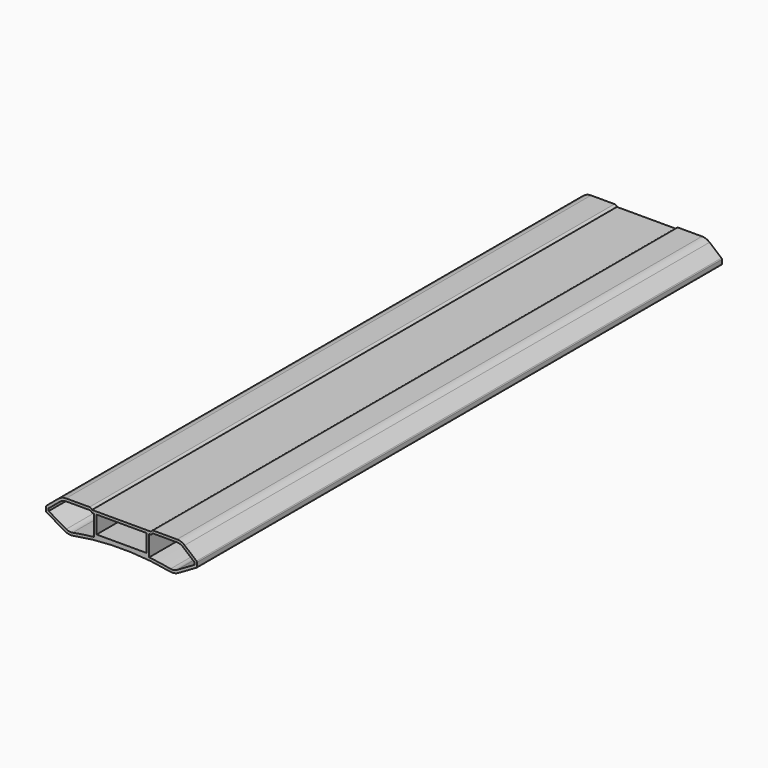
from build123d import *

# Parameters (mm, degrees)
F1_DEPTH    = 250
F2_W        = 38
F2_H        = 13.3740238536
F3_DEPTH    = 1200
F4_T1_DEPTH = 509.3674969976
F5_R        = 9
F6_R        = 1
F8_DEPTH    = 500.001


# Not quite as in the source:
# - a fillet or chamfer that OpenCascade refuses, or shapes differently, is made with other operations: its cross-section is extruded or revolved along the edge and cut away or added


with BuildPart() as f1:
    # F0 (on Front) → F1 (new body, symmetric)
    with BuildSketch(Plane.XZ):
        with BuildLine():
            Line((-57.5, 2.6740238536), (-40.1794919243, -7.3259761464))
            ThreePointArc((-40.1794919243, -7.3259761464), (0, -3.248431288), (40.1794919243, -7.3259761464))
            Line((40.1794919243, -7.3259761464), (57.5, 2.6740238536))
            Line((57.5, 2.6740238536), (57.5, 6.6740238536))
            Line((57.5, 6.6740238536), (45.5824640741, 16.6740238536))
            Line((45.5824640741, 16.6740238536), (22.5, 16.6740238536))
            Line((22.5, 16.6740238536), (22.5, 15.3740238536))
            Line((22.5, 15.3740238536), (0, 15.3740238536))
            Line((0, 15.3740238536), (-22.5, 15.3740238536))
            Line((-22.5, 15.3740238536), (-22.5, 16.6740238536))
            Line((-22.5, 16.6740238536), (-45.5824640741, 16.6740238536))
            Line((-45.5824640741, 16.6740238536), (-57.5, 6.6740238536))
            Line((-57.5, 6.6740238536), (-57.5, 2.6740238536))
        make_face()
    extrude(amount=F1_DEPTH, both=True)

    # F2 (on face) → F3 (cut)
    with BuildSketch(Plane.XZ.offset(250)):
        with Locations((0, 6.6870119268)):
            Rectangle(F2_W, F2_H)
    extrude(amount=-F3_DEPTH, mode=Mode.SUBTRACT)

    # F4: fillet of radius 2 on 2 edges, made by hand

    # F4_s2 → F4_t1 (cut)
    with BuildSketch(Plane.XZ.offset(-254.6837484988)):
        with BuildLine():
            ThreePointArc((-24.3734993995, 16.6740238536), (-23.2333239744, 16.3171915261), (-22.5, 15.3740238536))
            Line((-22.5, 15.3740238536), (-22.5, 16.6740238536))
            Line((-22.5, 16.6740238536), (-24.3734993995, 16.6740238536))
        make_face()
        with BuildLine():
            ThreePointArc((24.3734993995, 16.6740238536), (23.2333239744, 16.3171915261), (22.5, 15.3740238536))
            Line((22.5, 15.3740238536), (22.5, 16.6740238536))
            Line((22.5, 16.6740238536), (24.3734993995, 16.6740238536))
        make_face()
    extrude(amount=F4_T1_DEPTH, mode=Mode.SUBTRACT)

    # F5
    f5_edges = [f1.edges().sort_by_distance(p)[0] for p in [
        (45.582464, 0, 16.674024),
        (40.179492, 0, -7.325976),
        (-45.582464, 0, 16.674024),
        (-40.179492, 0, -7.325976),
    ]]
    fillet(f5_edges, radius=F5_R)

    # F6
    f6_edges = [f1.edges().sort_by_distance(p)[0] for p in [
        (-57.5, 0, 6.674024),
        (-57.5, 0, 2.674024),
        (57.5, 0, 6.674024),
        (57.5, 0, 2.674024),
    ]]
    fillet(f6_edges, radius=F6_R)

    # F7 (on face) → F8 (cut, through all)
    with BuildSketch(Plane.XZ.offset(250)):
        with BuildLine():
            ThreePointArc((-42.102269028, -3.9064590428), (-39.7790673217, -4.7446540804), (-37.3093701512, -4.7238460325))
            ThreePointArc((-37.3093701512, -4.7238460325), (-29.178978452, -3.3669982622), (-20.9999997169, -2.3429807302))
            Line((-20.9999997169, -2.3429807302), (-20.9999997169, 13.3740240708))
            Line((-20.9999997169, 13.3740240708), (-22.500000096, 13.3740240708))
            ThreePointArc((-22.500000096, 13.3740240708), (-23.2333241124, 14.3171915037), (-24.3734993995, 14.6740237251))
            Line((-24.3734993995, 14.6740237251), (-42.3067319657, 14.6740237251))
            ThreePointArc((-42.3067319657, 14.6740237251), (-44.700872925, 14.2518720783), (-46.8062451509, 13.036334857))
            Line((-46.8062451509, 13.036334857), (-55.4999998715, 5.7414084774))
            Line((-55.4999998715, 5.7414084774), (-55.4999998715, 3.8287244662))
            Line((-55.4999998715, 3.8287244662), (-42.102269028, -3.9064590428))
        make_face()
        with BuildLine():
            ThreePointArc((24.3734993995, 14.6740237251), (23.2333241124, 14.3171915037), (22.500000096, 13.3740240708))
            Line((22.500000096, 13.3740240708), (20.9999997169, 13.3740240708))
            Line((20.9999997169, 13.3740240708), (20.9999997169, -2.3429807302))
            ThreePointArc((20.9999997169, -2.3429807302), (29.178978452, -3.3669982622), (37.3093701512, -4.7238460325))
            ThreePointArc((37.3093701512, -4.7238460325), (39.7790673217, -4.7446540804), (42.102269028, -3.9064590428))
            Line((42.102269028, -3.9064590428), (55.4999998715, 3.8287244662))
            Line((55.4999998715, 3.8287244662), (55.4999998715, 5.7414084774))
            Line((55.4999998715, 5.7414084774), (46.8062451509, 13.036334857))
            ThreePointArc((46.8062451509, 13.036334857), (44.700872925, 14.2518720783), (42.3067319657, 14.6740237251))
            Line((42.3067319657, 14.6740237251), (24.3734993995, 14.6740237251))
        make_face()
    extrude(amount=-F8_DEPTH, mode=Mode.SUBTRACT)


solid = f1.part
